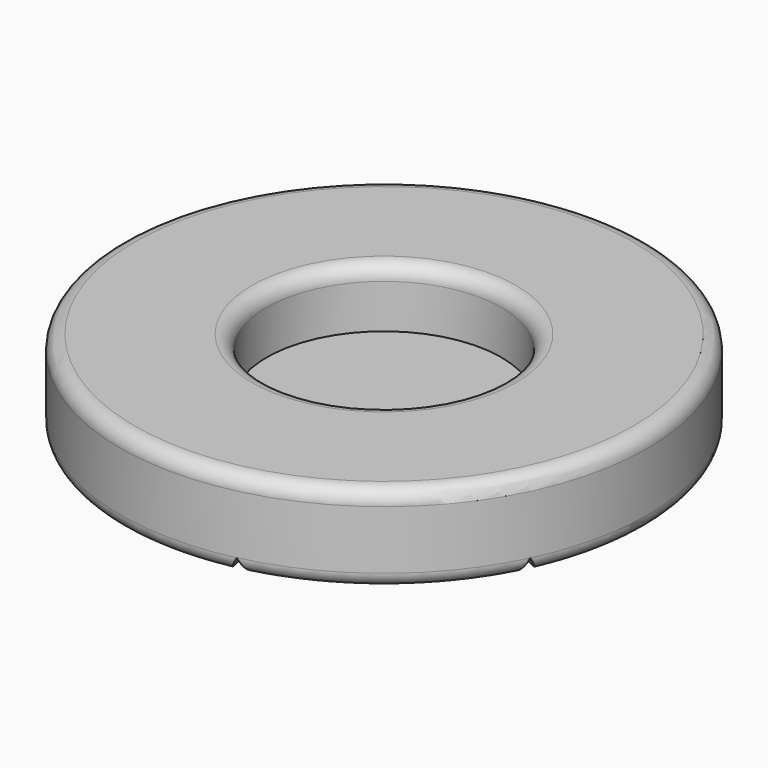
from build123d import *

# Parameters (mm, degrees)
F0_R            = 9
F0_R_2          = 4
F1_DEPTH        = 3
F2_R            = 4
F3_DEPTH        = 1
F4_R            = 0.5
F6_DEPTH        = 9.001
F6_COPIES_COUNT = 7
F10_R           = 0.5


# Not quite as in the source:
# - a pattern or mirror of a feature is missing from the dataset's text; its kind, count and spacing are read off the source's solid


with BuildPart() as f1:
    # F0 (on Top) → F1 (new body)
    with BuildSketch(Plane.XY):
        Circle(F0_R)
        Circle(F0_R_2, mode=Mode.SUBTRACT)
    extrude(amount=F1_DEPTH)

    # F2 (on face) → F3 (join)
    with BuildSketch(Plane(origin=(0, 0, 0), x_dir=(1, 0, 0), z_dir=(0, 0, -1))):
        Circle(F2_R)
    extrude(amount=-F3_DEPTH)

    # F4
    f4_edges = [f1.edges().sort_by_distance(p)[0] for p in [
        (-9, 0, 0),
        (-9, 0, 3),
    ]]
    fillet(f4_edges, radius=F4_R)

    # F5 (on Right) → F6 (cut, through all)
    with BuildSketch(Plane.YZ):
        Polygon((-0.2886751346, 0), (0.2886751346, 0), (0, 0.5), align=None)
    f6 = extrude(amount=-F6_DEPTH, mode=Mode.SUBTRACT)

    # F6_copies: F6 ×7 about axis
    f6_copies_axis = Axis((0, 0, 0), (0, 0, 1))
    for i in range(1, F6_COPIES_COUNT):
        add(f6.rotate(f6_copies_axis, i * 360 / F6_COPIES_COUNT), mode=Mode.SUBTRACT)

    # F7 (on Right) → F9 (revolve, cut)
    with BuildSketch(Plane.YZ):
        Polygon((4.5, 0.5), (4.2113248654, 0), (4.7886751346, 0), align=None)
    revolve(axis=Axis((0, 0, 0.5049179308), (0, 0, 1)), mode=Mode.SUBTRACT)

    # F10
    f10_edges = [f1.edges().sort_by_distance(p)[0] for p in [
        (-4, 0, 3),
    ]]
    fillet(f10_edges, radius=F10_R)


solid = f1.part
